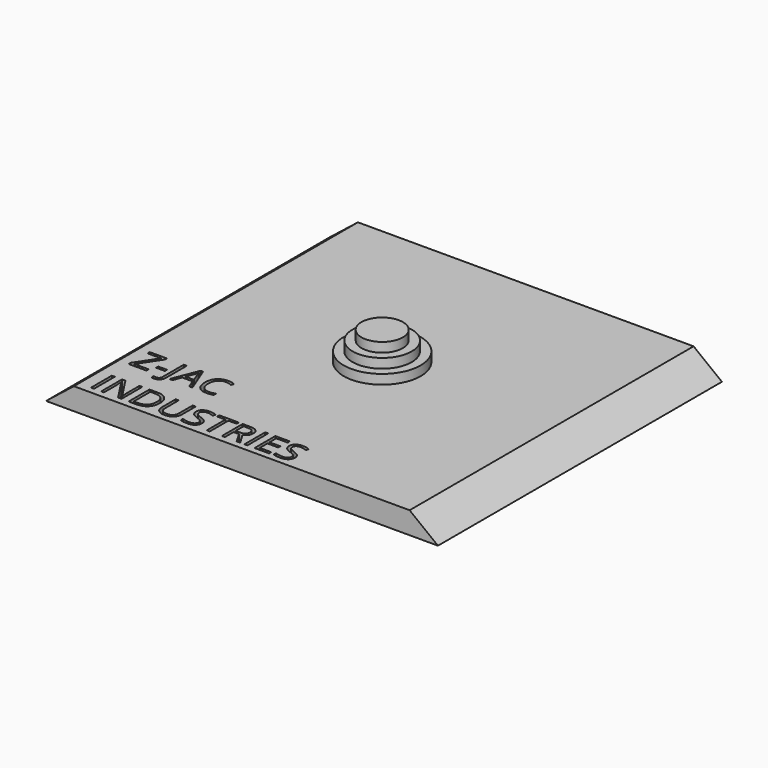
from build123d import *

# Parameters (mm, degrees)
F1_DEPTH     = 76.2
F3_R         = 8.255
F4_DEPTH     = 2.032
F5_R         = 6.35
F6_DEPTH     = 2.032
F7_R         = 4.445
F8_DEPTH     = 2.032
F9_TEXT_SIZE = 7.8204870483
F10_DEPTH    = 2.54


# Not quite as in the source:
# - Text() gives the source's letters only with a copy of the font that has no kerning and outlines rounded to 1/6400 em; it was checked with that copy


with BuildPart() as f1:
    # F0 (on Front) → F1 (new body)
    with BuildSketch(Plane.XZ):
        Polygon((-40.8264584839, 0), (-2.7264584839, 0), (43.2908311486, 0), (37.2120440006, 4.7297578818), (-34.8520304461, 4.7297578818), align=None)
    extrude(amount=F1_DEPTH)

    # F3 (on face) → F4 (join)
    with BuildSketch(Plane.XY.offset(4.7297578818)):
        with Locations((0, -37.0477512479)):
            Circle(F3_R)
    extrude(amount=F4_DEPTH)

    # F5 (on face) → F6 (join)
    with BuildSketch(Plane.XY.offset(6.7617578818)):
        with Locations((0, -37.0477512479)):
            Circle(F5_R)
    extrude(amount=F6_DEPTH)

    # F7 (on face) → F8 (join)
    with BuildSketch(Plane.XY.offset(8.7937578818)):
        with Locations((0, -37.0477512479)):
            Circle(F7_R)
    extrude(amount=F8_DEPTH)

    # F9 (on face) → F10 (cut)
    with BuildSketch(Plane.XY.offset(4.7297578818)):
        with Locations((-33.057782799, -64.1737473197)):
            Text('Z-JAC', F9_TEXT_SIZE, font='Open Sans', text_align=(TextAlign.LEFT, TextAlign.BOTTOM))
        with Locations((-33.057782799, -74.8096097054)):
            Text('INDUSTRIES', F9_TEXT_SIZE, font='Open Sans', text_align=(TextAlign.LEFT, TextAlign.BOTTOM))
    extrude(amount=-F10_DEPTH, mode=Mode.SUBTRACT)


solid = f1.part
